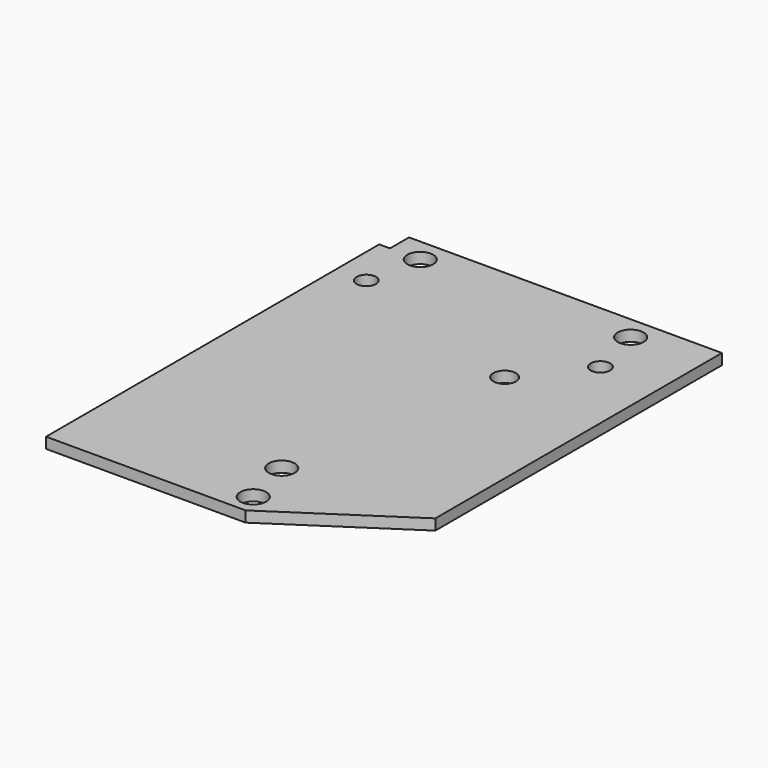
from build123d import *

# Parameters (mm, degrees)
F0_R     = 1.2
F0_R_2   = 0.9
F0_R_3   = 1.05
F1_DEPTH = 1


# Not quite as in the source:
# - a feature of the source that left no trace in its solid (it failed there, or was rolled back) is left out


with BuildPart() as f1:
    # F0 (on Top) → F1 (new body)
    with BuildSketch(Plane.XY):
        Polygon((27.5302478731, -17.7104764104), (27.5302478731, 15.4895235896), (-1.4697521269, 15.4895235896), (-1.4697521269, 13.2895235896), (-2.4697521269, 13.2895235896), (-2.4697521269, -22.3104764104), (-2.4697521269, -25.3104764104), (-1.4697521269, -25.3104764104), (16.0302478731, -25.3104764104), align=None)
        with Locations((15.1302478731, -23.3104764104)):
            Circle(F0_R, mode=Mode.SUBTRACT)
        with Locations((13.9302478731, -18.5104764104)):
            Circle(F0_R, mode=Mode.SUBTRACT)
        with Locations((0.3302478731, 8.2895235896)):
            Circle(F0_R_2, mode=Mode.SUBTRACT)
        with Locations((1.3302478731, 13.2895235896)):
            Circle(F0_R, mode=Mode.SUBTRACT)
        with Locations((17.6302478731, 2.6895235896)):
            Circle(F0_R_3, mode=Mode.SUBTRACT)
        with Locations((22.0302478731, 8.2895235896)):
            Circle(F0_R_2, mode=Mode.SUBTRACT)
        with Locations((20.8302478731, 13.2895235896)):
            Circle(F0_R, mode=Mode.SUBTRACT)
    extrude(amount=F1_DEPTH)


solid = f1.part
